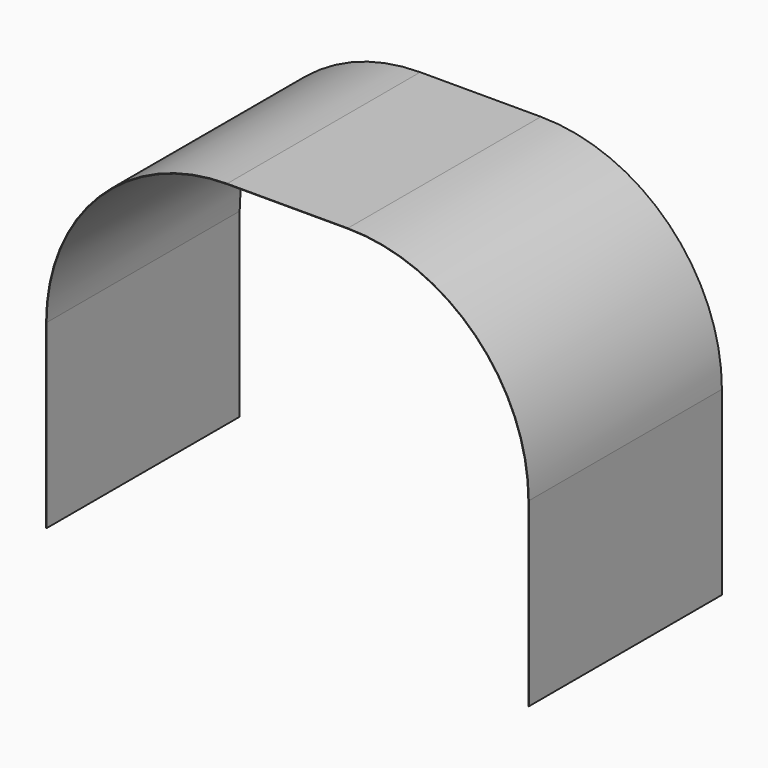
from build123d import *

# Parameters (mm, degrees)
F0_W     = 2000
F0_H     = 1500
F1_DEPTH = 500
F2_R     = 750
F4_DEPTH = 1000.001


# Not quite as in the source:
# - a feature names something its author has since deleted; it is built from what else it names


with BuildPart() as f1:
    # F0 (on Front) → F1 (new body, symmetric)
    with BuildSketch(Plane.XZ):
        with Locations((0, 750)):
            Rectangle(F0_W, F0_H)
    extrude(amount=F1_DEPTH, both=True)

    # F2
    f2_edges = [f1.edges().sort_by_distance(p)[0] for p in [
        (-1000, 0, 1500),
        (1000, 0, 1500),
    ]]
    fillet(f2_edges, radius=F2_R)

    # F3 (on face) → F4 (cut, through all)
    with BuildSketch(Plane.XZ.offset(500)):
        with BuildLine():
            ThreePointArc((-250, 1498), (-778.9158723275, 1278.9158723275), (-998, 750))
            Line((-998, 750), (-998, -0.5737363658))
            Line((-998, -0.5737363658), (998, -0.5742163858))
            Line((998, -0.5742163858), (998, 750))
            ThreePointArc((998, 750), (778.9158723275, 1278.9158723275), (250, 1498))
            Line((250, 1498), (-250, 1498))
        make_face()
    extrude(amount=-F4_DEPTH, mode=Mode.SUBTRACT)


solid = f1.part
